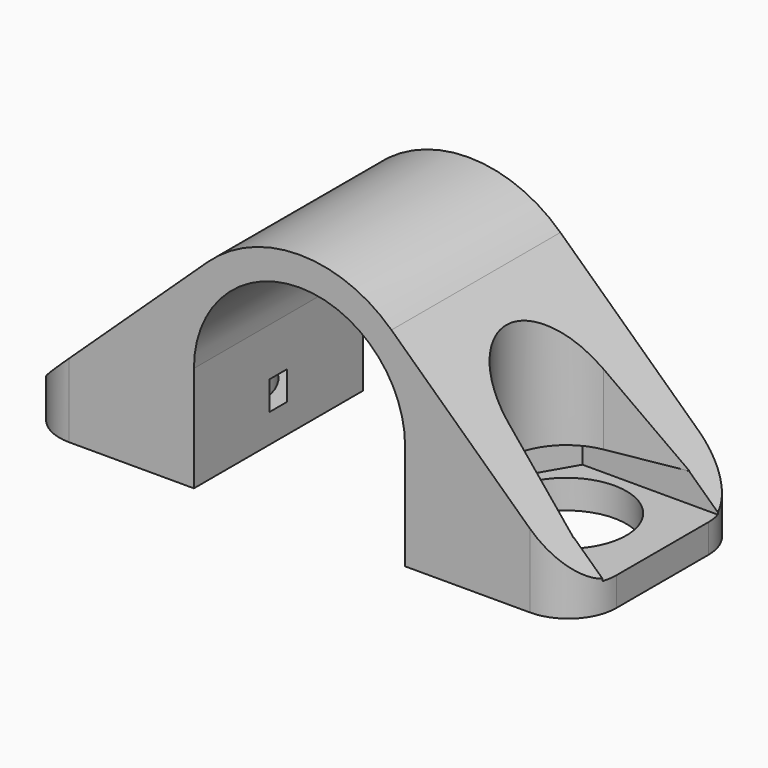
from build123d import *

# Parameters (mm, degrees)
F2_DEPTH     = 11
F5_DEPTH     = 3
F6_R         = 6.25
F7_DEPTH     = 25.001
F9_DEPTH     = 19.001
F10_T1_DEPTH = 28


# Not quite as in the source:
# - a fillet or chamfer that OpenCascade refuses, or shapes differently, is made with other operations: its cross-section is extruded or revolved along the edge and cut away or added
# - a pattern or mirror of a feature is missing from the dataset's text; its kind, count and spacing are read off the source's solid


with BuildPart() as f2:
    # F1 (on Front) → F2 (new body, symmetric)
    with BuildSketch(Plane.XZ):
        with BuildLine():
            ThreePointArc((-11, 11), (0, 22), (11, 11))
            Line((11, 11), (11, 0))
            Line((11, 0), (29, 0))
            Line((29, 0), (29, 3))
            Line((29, 3), (9.5759447935, 21.2127998763))
            ThreePointArc((9.5759447935, 21.2127998763), (0, 25), (-9.5759447935, 21.2127998763))
            Line((-9.5759447935, 21.2127998763), (-29, 3))
            Line((-29, 3), (-29, 0))
            Line((-29, 0), (-11, 0))
            Line((-11, 0), (-11, 11))
        make_face()
    extrude(amount=F2_DEPTH, both=True)

    # F4 (on plane+point) → F5 (cut)
    with BuildSketch(Plane.XY.offset(3)):
        Polygon((-10.3397459622, 0), (-14.6698729811, 7.5), (-37.1779240668, 7.5), (-37.1779240668, -7.5), (-14.6698729811, -7.5), align=None)
    f5 = extrude(amount=F5_DEPTH, mode=Mode.SUBTRACT)

    # F5_copies: F5 across plane
    add(f5.mirror(Plane(origin=(0, 0, 0), x_dir=(0, 0, 1), z_dir=(1, 0, 0))), mode=Mode.SUBTRACT)

    # F6 (on Top) → F7 (cut, through all)
    with BuildSketch(Plane.XY):
        with Locations((-19, 0)):
            Circle(F6_R)
    f7 = extrude(amount=F7_DEPTH, mode=Mode.SUBTRACT)

    # F7_copies: F7 across plane
    add(f7.mirror(Plane(origin=(0, 0, 0), x_dir=(0, 0, 1), z_dir=(1, 0, 0))), mode=Mode.SUBTRACT)

    # F8 (on face) → F9 (cut, through all)
    with BuildSketch(Plane(origin=(0, 0, 6), x_dir=(1, 0, 0), z_dir=(0, 0, -1))):
        with BuildLine():
            Line((-27, -7.75703217), (-17.9146988896, -6.1550484563))
            ThreePointArc((-17.9146988896, -6.1550484563), (-12.75, 0), (-17.9146988896, 6.1550484563))
            Line((-17.9146988896, 6.1550484563), (-27, 7.75703217))
            Line((-27, 7.75703217), (-27, -7.75703217))
        make_face()
    f9 = extrude(amount=-F9_DEPTH, mode=Mode.SUBTRACT)

    # F9_copies: F9 across plane
    add(f9.mirror(Plane(origin=(0, 0, 0), x_dir=(0, 0, 1), z_dir=(1, 0, 0))), mode=Mode.SUBTRACT)

    # F10: fillet of radius 5 on 4 edges, made by hand

    # F10_s2 → F10_t1 (cut)
    with BuildSketch(Plane.XY.offset(-12.5)):
        with BuildLine():
            ThreePointArc((-29, -6), (-27.5355339059, -9.5355339059), (-24, -11))
            Line((-24, -11), (-29, -11))
            Line((-29, -11), (-29, -6))
        make_face()
        with BuildLine():
            ThreePointArc((-29, 6), (-27.5355339059, 9.5355339059), (-24, 11))
            Line((-24, 11), (-29, 11))
            Line((-29, 11), (-29, 6))
        make_face()
        with BuildLine():
            ThreePointArc((29, -6), (27.5355339059, -9.5355339059), (24, -11))
            Line((24, -11), (29, -11))
            Line((29, -11), (29, -6))
        make_face()
        with BuildLine():
            ThreePointArc((29, 6), (27.5355339059, 9.5355339059), (24, 11))
            Line((24, 11), (29, 11))
            Line((29, 11), (29, 6))
        make_face()
    extrude(amount=F10_T1_DEPTH, mode=Mode.SUBTRACT)


solid = f2.part
